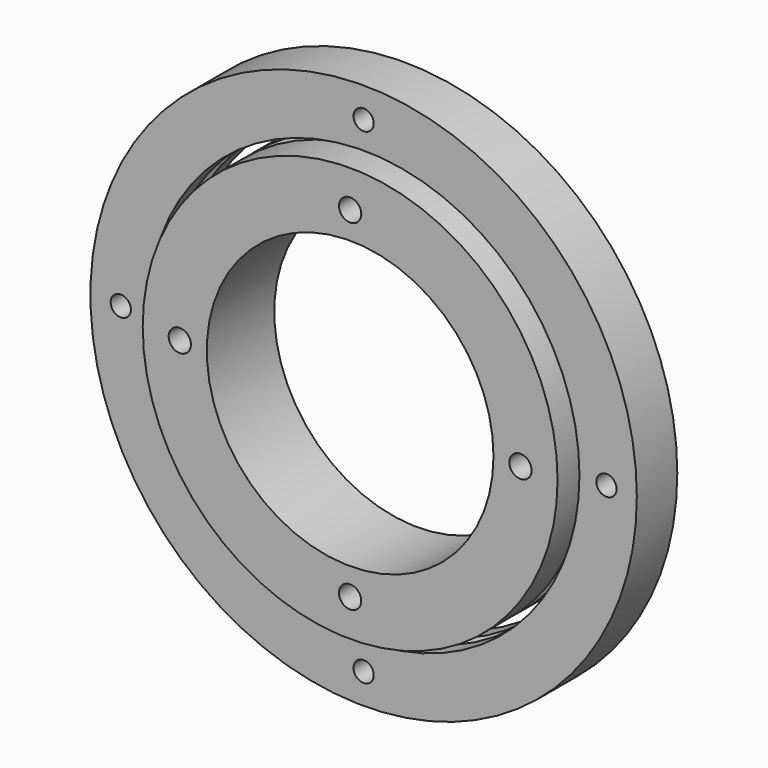
from build123d import *

# Parameters (mm, degrees)
F0_R            = 81
F0_R_2          = 64
F1_DEPTH        = 7.5
F2_R            = 61.5
F2_R_2          = 42.5
F3_DEPTH        = 12.5
F4_R            = 2.5
F8_D            = 6.6
F8_CBORE_D      = 10
F8_CBORE_DEPTH  = 5
F8_COPIES_COUNT = 4
F9_D            = 6
F9_COPIES_COUNT = 4


# Not quite as in the source:
# - a pattern or mirror of a feature is missing from the dataset's text; its kind, count and spacing are read off the source's solid


with BuildPart() as f1:
    # F0 (on Front) → F1 (new body, symmetric)
    with BuildSketch(Plane.XZ):
        Circle(F0_R)
        Circle(F0_R_2, mode=Mode.SUBTRACT)
    extrude(amount=F1_DEPTH, both=True)


with BuildPart() as f3:
    # F2 (on Front) → F3 (new body, symmetric)
    with BuildSketch(Plane.XZ):
        Circle(F2_R)
        Circle(F2_R_2, mode=Mode.SUBTRACT)
    extrude(amount=F3_DEPTH, both=True)


with BuildPart() as f5_tool:
    # F4 (on Right) → F5 (revolve)
    with BuildSketch(Plane.YZ):
        with Locations((0, 62.75)):
            Circle(F4_R)
    revolve(axis=Axis((0, 0, 0), (0, 1, 0)))


with BuildPart() as f1_1:
    add(f1.part)

    # F5: cut by f5_tool
    add(f5_tool.part, mode=Mode.SUBTRACT)

    # F9 (through all)
    with Locations(Plane.XZ.offset(7.5)):
        with Locations((0, 72)):
            f9 = Hole(F9_D / 2)

    # F9_copies: F9 ×4 about axis
    f9_copies_axis = Axis((0, 0, 0), (0, 1, 0))
    for i in range(1, F9_COPIES_COUNT):
        add(f9.rotate(f9_copies_axis, i * 360 / F9_COPIES_COUNT), mode=Mode.SUBTRACT)


with BuildPart() as f3_1:
    add(f3.part)

    # F5: cut by f5_tool
    add(f5_tool.part, mode=Mode.SUBTRACT)

    # F8 (through all)
    with Locations(Plane(origin=(0, 12.5, 0), x_dir=(-1, 0, 0), z_dir=(0, 1, 0))):
        with Locations((0, 50.5)):
            f8 = CounterBoreHole(F8_D / 2, F8_CBORE_D / 2, F8_CBORE_DEPTH)

    # F8_copies: F8 ×4 about axis
    f8_copies_axis = Axis((0, 0, 0), (0, 1, 0))
    for i in range(1, F8_COPIES_COUNT):
        add(f8.rotate(f8_copies_axis, i * 360 / F8_COPIES_COUNT), mode=Mode.SUBTRACT)


solid = Compound([f1_1.part, f3_1.part])
